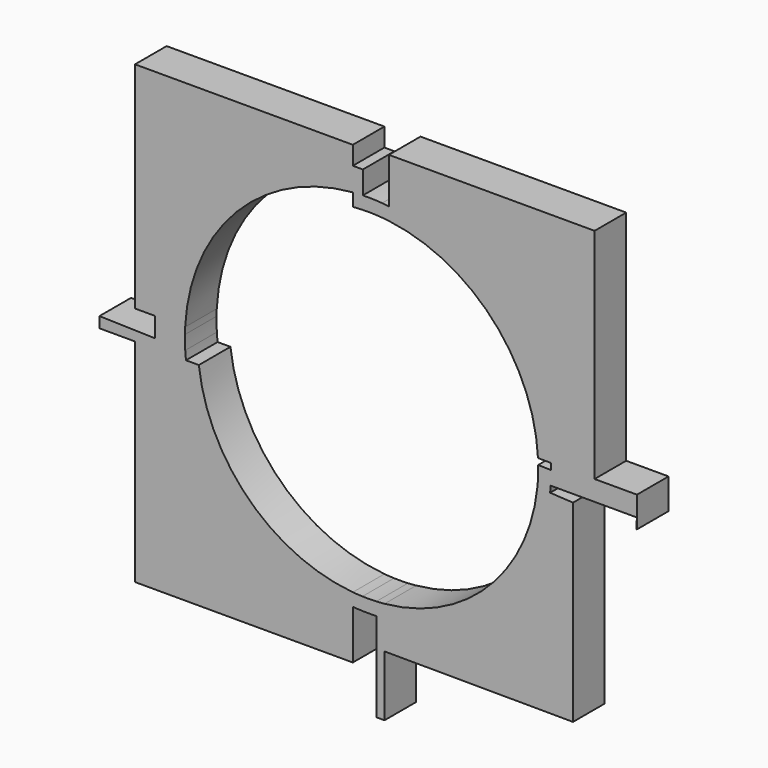
from build123d import *

# Parameters (mm, degrees)
F1_DEPTH = 8


with BuildPart() as f1:
    # F0 (on Front) → F1 (new body)
    with BuildSketch(Plane.XZ):
        Polygon((-47.1591800451, -3.9871255867), (-47.1591800451, -46.8671731651), (-3.0660768971, -46.8671731651), (-3.0660768971, -42.9581068456), (-43.1017912924, -42.9581068456), (-43.1017912924, -3.9871255867), align=None)
        Polygon((-54.3611483469, -3.9871255867), (-47.1591800451, -3.9871255867), (-43.1017912924, -3.9871255867), (-43.1017912924, -2.1041460184), (-54.3611483469, -1.8037535483), align=None)
        with BuildLine():
            Line((-43.1017912924, -42.9581068456), (-3.0660768971, -42.9581068456))
            Line((-3.0660768971, -42.9581068456), (-3.0660768971, -36.9308893154))
            ThreePointArc((-3.0660768971, -36.9308893154), (-25.8747586881, -26.5290081986), (-36.8428316328, -3.9871255867))
            Line((-36.8428316328, -3.9871255867), (-43.1017912924, -3.9871255867))
            Line((-43.1017912924, -3.9871255867), (-43.1017912924, -42.9581068456))
        make_face()
        with BuildLine():
            Line((-43.1017912924, -2.1041460184), (-43.1017912924, -3.9871255867))
            Line((-43.1017912924, -3.9871255867), (-36.8428316328, -3.9871255867))
            ThreePointArc((-36.8428316328, -3.9871255867), (-36.9256932446, -3.12803318), (-36.9885254852, -2.2672440539))
            Line((-36.9885254852, -2.2672440539), (-43.1017912924, -2.1041460184))
        make_face()
        with BuildLine():
            ThreePointArc((-36.8428316328, -3.9871255867), (-25.8747586881, -26.5290081986), (-3.0660768971, -36.9308893154))
            Line((-3.0660768971, -36.9308893154), (-3.0660768971, -34.3354971844))
            ThreePointArc((-3.0660768971, -34.3354971844), (-24.0459151958, -24.7006306971), (-34.2407655288, -3.9871255867))
            Line((-34.2407655288, -3.9871255867), (-36.8428316328, -3.9871255867))
        make_face()
        with BuildLine():
            Line((-3.0660768971, -34.3354971844), (-3.0660768971, -36.9308893154))
            ThreePointArc((-3.0660768971, -36.9308893154), (-2.0633689571, -37.0004583987), (-1.0591430979, -37.0428080613))
            Line((-1.0591430979, -37.0428080613), (-1.1211578882, -34.4538851137))
            ThreePointArc((-1.1211578882, -34.4538851137), (-2.0944540368, -34.4084358367), (-3.0660768971, -34.3354971844))
        make_face()
        with BuildLine():
            Line((-43.1017912924, 0.534063729), (-43.1017912924, -2.1041460184))
            Line((-43.1017912924, -2.1041460184), (-36.9885254852, -2.2672440539))
            ThreePointArc((-36.9885254852, -2.2672440539), (-37.0477983113, -0.867210155), (-37.0540981418, 0.534063729))
            Line((-37.0540981418, 0.534063729), (-43.1017912924, 0.534063729))
        make_face()
        with BuildLine():
            Line((-1.1211578882, -34.4538851137), (-1.0591430979, -37.0428080613))
            ThreePointArc((-1.0591430979, -37.0428080613), (0.3177187709, -37.0565846774), (1.6941420035, -37.0192017207))
            Line((1.6941420035, -37.0192017207), (1.6941420035, -34.4304672828))
            ThreePointArc((1.6941420035, -34.4304672828), (0.2867312292, -34.4709294862), (-1.1211578882, -34.4538851137))
        make_face()
        with BuildLine():
            Line((-43.1017912924, 1.8888709601), (-43.1017912924, 0.534063729))
            Line((-43.1017912924, 0.534063729), (-37.0540981418, 0.534063729))
            ThreePointArc((-37.0540981418, 0.534063729), (-37.0381326331, 1.2116700136), (-37.0097768119, 1.8888709601))
            Line((-37.0097768119, 1.8888709601), (-43.1017912924, 1.8888709601))
        make_face()
        with BuildLine():
            ThreePointArc((3.3580851741, -36.9054830226), (2.5267534207, -36.9717044551), (1.6941420035, -37.0192017207))
            Line((1.6941420035, -37.0192017207), (1.6941420035, -55.0743453205))
            Line((1.6941420035, -55.0743453205), (3.3580851741, -55.0743453205))
            Line((3.3580851741, -55.0743453205), (3.3580851741, -46.8671731651))
            Line((3.3580851741, -46.8671731651), (3.3580851741, -42.7945544943))
            Line((3.3580851741, -42.7945544943), (3.3580851741, -36.9054830226))
        make_face()
        with BuildLine():
            Line((1.6941420035, -34.4304672828), (1.6941420035, -37.0192017207))
            ThreePointArc((1.6941420035, -37.0192017207), (2.5267534207, -36.9717044551), (3.3580851741, -36.9054830226))
            Line((3.3580851741, -36.9054830226), (3.3580851741, -34.3081689748))
            ThreePointArc((3.3580851741, -34.3081689748), (2.5268535934, -34.3793863435), (1.6941420035, -34.4304672828))
        make_face()
        Polygon((-47.1591800451, 1.8888709601), (-43.1017912924, 1.8888709601), (-43.1017912924, 41.1945804954), (-43.1017912924, 41.6629081592), (-3.0660768971, 41.6629081592), (-3.0660768971, 45.4071350396), (-47.1591800451, 45.4071350396), align=None)
        with BuildLine():
            Line((-43.1017912924, 41.1945804954), (-43.1017912924, 1.8888709601))
            Line((-43.1017912924, 1.8888709601), (-37.0097768119, 1.8888709601))
            ThreePointArc((-37.0097768119, 1.8888709601), (-26.6177436164, 25.7834663678), (-3.0660768971, 36.9308893154))
            Line((-3.0660768971, 36.9308893154), (-3.0660768971, 41.6629081592))
            Line((-3.0660768971, 41.6629081592), (-43.1017912924, 41.6629081592))
            Line((-43.1017912924, 41.6629081592), (-43.1017912924, 41.1945804954))
        make_face()
        with BuildLine():
            ThreePointArc((36.8810945474, -3.6161136812), (26.1121317389, -26.295398632), (3.3580851741, -36.9054830226))
            Line((3.3580851741, -36.9054830226), (3.3580851741, -42.7945544943))
            Line((3.3580851741, -42.7945544943), (41.5107160807, -42.9581068456))
            Line((41.5107160807, -42.9581068456), (41.5107160807, -3.876257455))
            Line((41.5107160807, -3.876257455), (36.8810945474, -3.6161136813))
        make_face()
        with BuildLine():
            Line((3.3580851741, -34.3081689748), (3.3580851741, -36.9054830226))
            ThreePointArc((3.3580851741, -36.9054830226), (26.1121317389, -26.295398632), (36.8810945474, -3.6161136812))
            Line((36.8810945474, -3.6161136813), (34.2969386269, -3.4709069795))
            ThreePointArc((34.2969386269, -3.4709069795), (24.3353526008, -24.4155239189), (3.3580851741, -34.3081689748))
        make_face()
        with BuildLine():
            Line((34.2969386269, -3.4709069795), (36.8810945474, -3.6161136813))
            ThreePointArc((36.8810945474, -3.6161136812), (36.9391000222, -2.9655189628), (36.9856296892, -2.3140029516))
            Line((36.9856296892, -2.3140029516), (34.3943685039, -2.3140029516))
            ThreePointArc((34.3943685039, -2.3140029516), (34.3505243856, -2.8928651668), (34.2969386269, -3.4709069795))
        make_face()
        with BuildLine():
            ThreePointArc((-1.0392403929, 37.0433717765), (-2.0534289831, 37.0010113724), (-3.0660768971, 36.9308893154))
            Line((-3.0660768971, 36.9308893154), (-3.0660768971, 34.3354971844))
            ThreePointArc((-3.0660768971, 34.3354971844), (-2.0535493927, 34.4109013153), (-1.0392403929, 34.4564532976))
            Line((-1.0392403929, 34.4564532976), (-1.0392403929, 37.0433717765))
        make_face()
        with BuildLine():
            Line((-3.0660768971, 41.6629081592), (-3.0660768971, 36.9308893154))
            ThreePointArc((-3.0660768971, 36.9308893154), (-2.0534289831, 37.0010113724), (-1.0392403929, 37.0433717765))
            Line((-1.0392403929, 37.0433717765), (-1.0392403929, 41.6629081592))
            Line((-1.0392403929, 41.6629081592), (-3.0660768971, 41.6629081592))
        make_face()
        with BuildLine():
            Line((34.3943685039, -2.3140029516), (36.9856296892, -2.3140029516))
            ThreePointArc((36.9856296892, -2.3140029516), (37.0398630305, -1.157566349), (37.0579466939, 0))
            ThreePointArc((37.0579466939, 0), (37.0571653007, 0.2406512887), (37.0548211541, 0.4812924287))
            Line((37.0548211541, 0.4812924287), (34.4676887508, 0.5528350755))
            ThreePointArc((34.4676887508, 0.5528350755), (34.4710136618, 0.2764264252), (34.4721219892, 0))
            ThreePointArc((34.4721219892, 0), (34.4526781343, -1.1576544459), (34.3943685039, -2.3140029516))
        make_face()
        with BuildLine():
            ThreePointArc((37.0579466939, 0), (37.0398630305, -1.157566349), (36.9856296892, -2.3140029516))
            Line((36.9856296892, -2.3140029516), (54.4263494667, -2.3140029516))
            Line((54.4263494667, -2.3140029516), (54.4593664818, 0))
            Line((54.4593664818, 0), (45.8812378347, 0.2372132275))
            Line((45.8812378347, 0.2372132275), (37.0548211541, 0.4812924287))
            ThreePointArc((37.0548211541, 0.4812924287), (37.0571653007, 0.2406512887), (37.0579466939, 0))
        make_face()
        with BuildLine():
            ThreePointArc((2.8755131643, 36.9462154653), (0.919420611, 37.0465393648), (-1.0392403929, 37.0433717765))
            Line((-1.0392403929, 37.0433717765), (-1.0392403929, 34.4564532976))
            ThreePointArc((-1.0392403929, 34.4564532976), (0.9196211301, 34.4598533284), (2.8755131643, 34.351981289))
            Line((2.8755131643, 34.351981289), (2.8755131643, 36.9462154653))
        make_face()
        Polygon((54.4593664818, 0), (54.4263494667, -2.3140029516), (54.3960799696, -4.4354456477), (54.4593664818, -4.4354456477), align=None)
        with BuildLine():
            ThreePointArc((4.2341067456, 36.8152652202), (3.5554128885, 36.886995708), (2.8755131643, 36.9462154653))
            Line((2.8755131643, 36.9462154653), (2.8755131643, 34.351981289))
            ThreePointArc((2.8755131643, 34.351981289), (3.555507773, 34.2882714484), (4.2341067456, 34.2111025035))
            Line((4.2341067456, 34.2111025035), (4.2341067456, 36.8152652202))
        make_face()
        with BuildLine():
            ThreePointArc((37.0162491765, 1.7574726371), (37.0410316266, 1.119548661), (37.0548211541, 0.4812924287))
            Line((37.0548211541, 0.4812924287), (45.8812378347, 0.2372132275))
            Line((45.8812378347, 0.2372132275), (45.8812378347, 1.7574726371))
            Line((45.8812378347, 1.7574726371), (41.5107160807, 1.7574726371))
            Line((41.5107160807, 1.7574726371), (37.0162491765, 1.7574726371))
        make_face()
        Polygon((45.8812378347, 0.2372132275), (54.4593664818, 0), (54.4593664818, 1.7574726371), (45.8812378347, 1.7574726371), align=None)
        with BuildLine():
            ThreePointArc((37.0162491765, 1.7574726371), (27.0676960808, 25.3106942229), (4.2341067456, 36.8152652202))
            Line((4.2341067456, 36.8152652202), (4.2341067456, 34.2111025035))
            ThreePointArc((4.2341067456, 34.2111025035), (25.2385711785, 23.4806669264), (34.427292725, 1.7574726371))
            Line((34.427292725, 1.7574726371), (37.0162491765, 1.7574726371))
        make_face()
        with BuildLine():
            Line((4.2341067456, 41.2198267877), (4.2341067456, 36.8152652202))
            ThreePointArc((4.2341067456, 36.8152652202), (27.0676960808, 25.3106942229), (37.0162491765, 1.7574726371))
            Line((37.0162491765, 1.7574726371), (41.5107160807, 1.7574726371))
            Line((41.5107160807, 1.7574726371), (41.5107160807, 41.2198267877))
            Line((41.5107160807, 41.2198267877), (4.2341067456, 41.2198267877))
        make_face()
        Polygon((4.2341067456, 45.9911525249), (4.2341067456, 41.2198267877), (41.5107160807, 41.2198267877), (41.5107160807, 1.7574726371), (45.8812378347, 1.7574726371), (45.8812378347, 45.9911525249), align=None)
    extrude(amount=F1_DEPTH)


solid = f1.part
